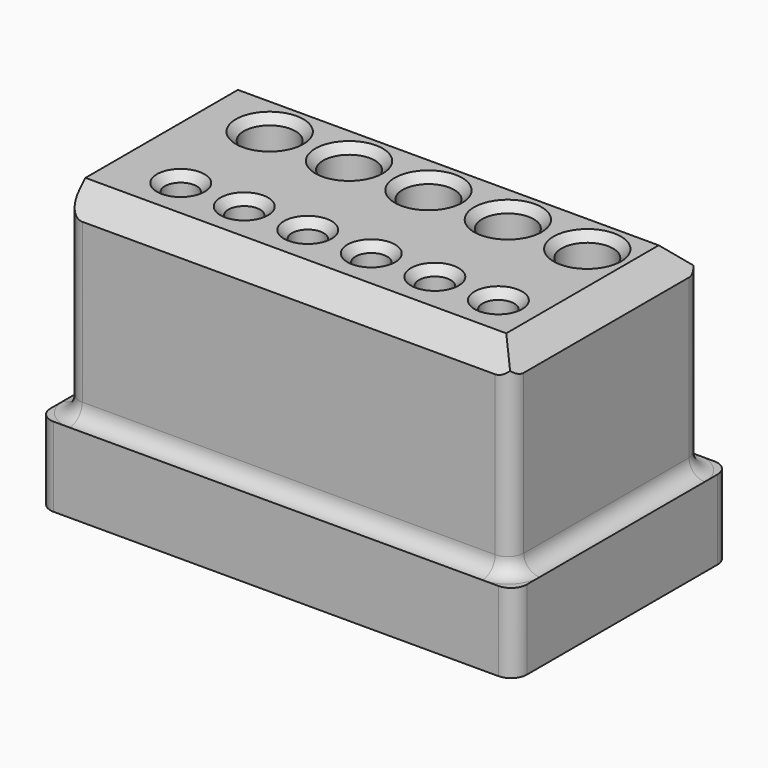
from build123d import *

# Parameters (mm, degrees)
F0_W      = 60
F0_H      = 34
F0_W_2    = 56
F0_H_2    = 30
F1_DEPTH  = 10
F2_DEPTH  = 35
F3_R      = 2
F3_R_2    = 3.25
F4_DEPTH  = 22
F5_SIZE   = 3
F6_SIZE   = 1
F7_R      = 2
F8_R      = 1.99999
F9_W      = 52
F9_H      = 24
F10_DEPTH = 9


# Not quite as in the source:
# - a fillet or chamfer is up to 0.001 mm smaller than in the source, because OpenCascade refuses the exact size


with BuildPart() as f1:
    # F0 (on Top) → F1 (new body)
    with BuildSketch(Plane.XY):
        Rectangle(F0_W, F0_H)
        Rectangle(F0_W_2, F0_H_2, mode=Mode.SUBTRACT)
        Rectangle(F0_W_2, F0_H_2)
    extrude(amount=F1_DEPTH)

    # F0 (on Top) → F2 (join)
    with BuildSketch(Plane.XY):
        Rectangle(F0_W_2, F0_H_2)
    extrude(amount=F2_DEPTH)

    # F3 (on face) → F4 (cut)
    with BuildSketch(Plane.XY.offset(35)):
        with Locations((-20, -7)):
            Circle(F3_R)
        with Locations((-12, -7)):
            Circle(F3_R)
        with Locations((-4, -7)):
            Circle(F3_R)
        with Locations((4, -7)):
            Circle(F3_R)
        with Locations((12, -7)):
            Circle(F3_R)
        with Locations((20, -7)):
            Circle(F3_R)
        with Locations((-20, 7)):
            Circle(F3_R_2)
        with Locations((-10, 7)):
            Circle(F3_R_2)
        with Locations((0, 7)):
            Circle(F3_R_2)
        with Locations((10, 7)):
            Circle(F3_R_2)
        with Locations((20, 7)):
            Circle(F3_R_2)
    extrude(amount=-F4_DEPTH, mode=Mode.SUBTRACT)

    # F5
    f5_edges = [f1.edges().sort_by_distance(p)[0] for p in [
        (0, 15, 35),
        (28, 0, 35),
        (0, -15, 35),
    ]]
    chamfer(f5_edges, length=F5_SIZE)

    # F6
    f6_edges = [f1.edges().sort_by_distance(p)[0] for p in [
        (-16.75, 7, 24),
        (-23.25, 7, 35),
        (-23.25, 7, 13),
        (-13.25, 7, 35),
        (-3.25, 7, 35),
        (6.75, 7, 35),
        (16.75, 7, 35),
        (-22, -7, 35),
        (-14, -7, 35),
        (-6, -7, 35),
        (2, -7, 35),
        (10, -7, 35),
        (18, -7, 35),
    ]]
    chamfer(f6_edges, length=F6_SIZE)

    # F7
    f7_edges = [f1.edges().sort_by_distance(p)[0] for p in [
        (28, -15, 21),
        (-28, -15, 21),
        (28, 15, 21),
        (-28, 15, 21),
    ]]
    fillet(f7_edges, radius=F7_R)

    # F8 (radius 2 in the source; OpenCascade refuses exactly that, so slightly less here)
    f8_edges = [f1.edges().sort_by_distance(p)[0] for p in [
        (-30, -17, 5),
        (0, -15, 10),
        (30, -17, 5),
        (30, 17, 5),
        (-30, 17, 5),
    ]]
    fillet(f8_edges, radius=F8_R)


with BuildPart() as f10:
    # F9 (on face) → F10 (new body)
    with BuildSketch(Plane.XY):
        Rectangle(F9_W, F9_H)
    extrude(amount=F10_DEPTH)


solid = Compound([f1.part, f10.part])
